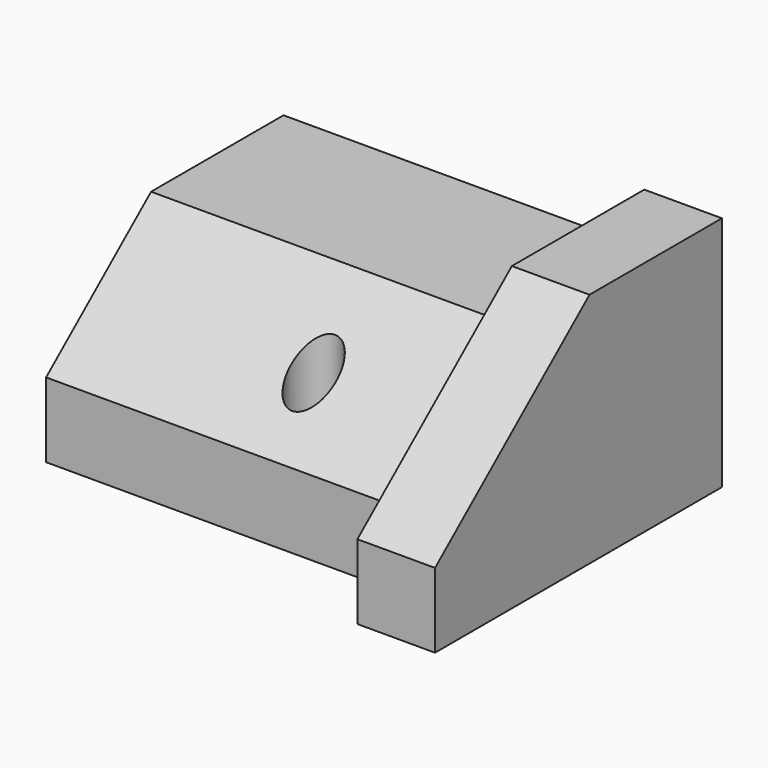
from build123d import *

# Parameters (mm, degrees)
F0_W        = 72.4030919373
F0_H        = 90.3663933277
F2_DEPTH    = 22.098
F1_W        = 15.5804120004
F1_H        = 90.3663933277
F3_DEPTH    = 32.512
F4_T1_DEPTH = 219.7018507435
F5_T1_DEPTH = 310.1779296127
F6_R        = 4.5271504528
F7_DEPTH    = 71.9636861302
F8_DEPTH    = 14.986


# Not quite as in the source:
# - a fillet or chamfer that OpenCascade refuses, or shapes differently, is made with other operations: its cross-section is extruded or revolved along the edge and cut away or added


with BuildPart() as f2:
    # F0 (on Top) → F2 (new body)
    with BuildSketch(Plane.XY):
        with Locations((-7.7902060002, 0)):
            Rectangle(F0_W, F0_H)
    extrude(amount=F2_DEPTH)

    # F1 (on face) → F3 (join)
    with BuildSketch(Plane.XY):
        with Locations((36.2015459687, 0)):
            Rectangle(F1_W, F1_H)
    extrude(amount=F3_DEPTH)

    # F4: chamfer of 57.15 x 47.9545439218 on 1 edges, made by hand

    # F4_s2 → F4_t1 (cut)
    with BuildSketch(Plane.YZ.offset(-191.290510775)):
        Polygon((11.9668033361, 22.098), (-45.1831966639, -25.8565439218), (-45.1831966639, 22.098), align=None)
    extrude(amount=F4_T1_DEPTH, mode=Mode.SUBTRACT)

    # F5: chamfer of 57.15 x 47.9545439218 on 1 edges, made by hand

    # F5_s2 → F5_t1 (cut)
    with BuildSketch(Plane.YZ.offset(-118.8874188377)):
        Polygon((11.9668033361, 32.512), (-45.1831966639, -15.4425439218), (-45.1831966639, 32.512), align=None)
    extrude(amount=F5_T1_DEPTH, mode=Mode.SUBTRACT)

    # F6 (on face) → F7 (cut, through all)
    with BuildSketch(Plane(origin=(0, 45.1831966639, 0), x_dir=(-1, 0, 0), z_dir=(0, 1, 0))):
        with Locations((0, 10.1730925962)):
            Circle(F6_R)
    extrude(amount=-F7_DEPTH, mode=Mode.SUBTRACT)

    # F8 (add): faces of the model
    f8_faces = [f2.faces().sort_by_distance(p)[0] for p in [
        (-7.7902060002, 28.575, 22.098),
        (-8.1168519447, -1.1571124664, 11.0857270906),
        (36.2015459687, -7.4063430651, 16.256),
        (36.2015459687, 28.575, 32.512),
    ]]
    extrude(f8_faces, amount=F8_DEPTH, dir=(0, 0, 1))


solid = f2.part
